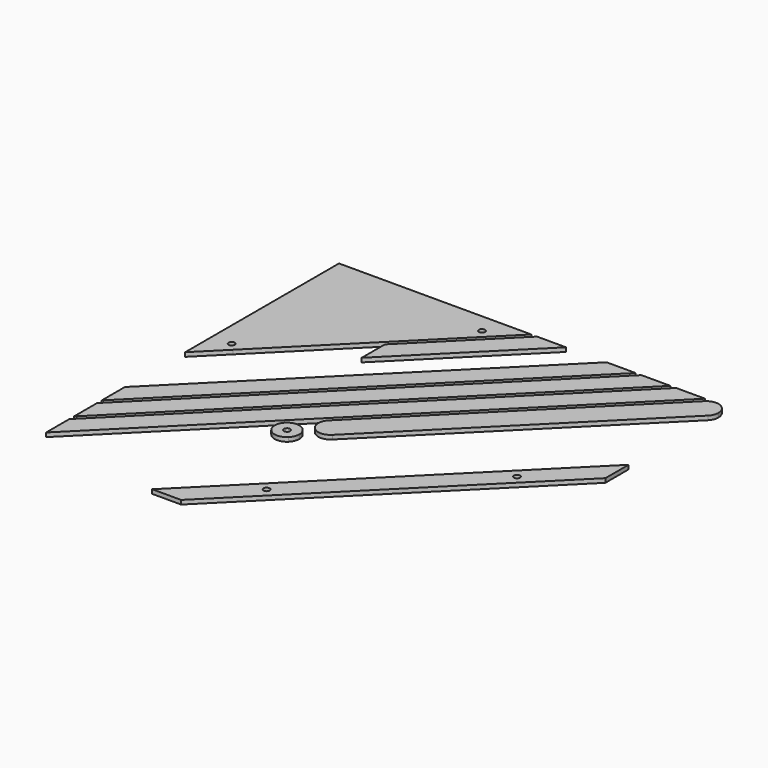
from build123d import *

# Parameters (mm, degrees)
F0_R     = 9.525
F1_DEPTH = 6.35


with BuildPart() as f1:
    # F0 (on Top) → F1 (new body, symmetric)
    with BuildSketch(Plane.XY):
        Polygon((-115.17049, 603.25), (-603.25, 603.25), (-603.25, 97.209977), (-603.25, 7.407416), (-520.854856, 89.802561), (-89.802561, 520.854855), (-7.407416, 603.25), align=None)
        with BuildLine():
            ThreePointArc((-511.555495, 112.253202), (-513.97232, 100.103002), (-520.854856, 89.802561))
            ThreePointArc((-520.854856, 89.802561), (-572.63867, 124.403401), (-511.555495, 112.253202))
        make_face(mode=Mode.SUBTRACT)
        with BuildLine():
            ThreePointArc((-80.503202, 543.305495), (-82.920026, 531.155296), (-89.802561, 520.854855))
            ThreePointArc((-89.802561, 520.854855), (-141.586377, 555.455694), (-80.503202, 543.305495))
        make_face(mode=Mode.SUBTRACT)
        with BuildLine():
            ThreePointArc((-511.555495, 112.253202), (-572.63867, 124.403401), (-520.854856, 89.802561))
            ThreePointArc((-520.854856, 89.802561), (-513.97232, 100.103002), (-511.555495, 112.253202))
        make_face()
        with Locations((-543.305495, 112.253202)):
            Circle(F0_R, mode=Mode.SUBTRACT)
        with BuildLine():
            ThreePointArc((-80.503202, 543.305495), (-141.586377, 555.455694), (-89.802561, 520.854855))
            ThreePointArc((-89.802561, 520.854855), (-82.920026, 531.155296), (-80.503202, 543.305495))
        make_face()
        with Locations((-112.253202, 543.305495)):
            Circle(F0_R, mode=Mode.SUBTRACT)
    extrude(amount=F1_DEPTH, both=True)


with BuildPart() as f1b:
    # F0 (on Top) → F1, piece 2 (new body, symmetric)
    with BuildSketch(Plane.XY):
        Polygon((-603.25, -226.079243), (-603.25, -315.881804), (-178.032283, 109.335913), (-222.933563, 154.237194), align=None)
        Polygon((-222.933563, 154.237194), (-178.032283, 109.335913), (315.881804, 603.25), (226.079243, 603.25), align=None)
    extrude(amount=F1_DEPTH, both=True)


with BuildPart() as f1c:
    # F0 (on Top) → F1, piece 3 (new body, symmetric)
    with BuildSketch(Plane.XY):
        Polygon((333.842316, 603.25), (-603.25, -333.842316), (-603.25, -423.644878), (423.644878, 603.25), align=None)
    extrude(amount=F1_DEPTH, both=True)


with BuildPart() as f1d:
    # F0 (on Top) → F1, piece 4 (new body, symmetric)
    with BuildSketch(Plane.XY):
        Polygon((-603.25, -441.60539), (-603.25, -531.407951), (531.407951, 603.25), (441.60539, 603.25), align=None)
    extrude(amount=F1_DEPTH, both=True)


with BuildPart() as f1e:
    # F0 (on Top) → F1, piece 5 (new body, symmetric)
    with BuildSketch(Plane.XY):
        with BuildLine():
            ThreePointArc((592.090768, 592.090768), (579.730239, 600.34981), (565.15, 603.25))
            ThreePointArc((565.15, 603.25), (550.569761, 600.34981), (538.209232, 592.090768))
            Line((538.209232, 592.090768), (-108.369209, -54.487672))
            ThreePointArc((-108.369209, -54.487672), (-119.528441, -81.428441), (-108.369209, -108.369209))
            Line((-108.369209, -108.369209), (592.090768, 592.090768))
        make_face()
        with BuildLine():
            ThreePointArc((592.090768, 538.209232), (600.34981, 550.569761), (603.25, 565.15))
            ThreePointArc((603.25, 565.15), (600.34981, 579.730239), (592.090768, 592.090768))
            Line((592.090768, 592.090768), (-108.369209, -108.369209))
            ThreePointArc((-108.369209, -108.369209), (-81.428441, -119.528441), (-54.487672, -108.369209))
            Line((-54.487672, -108.369209), (592.090768, 538.209232))
        make_face()
    extrude(amount=F1_DEPTH, both=True)


with BuildPart() as f1f:
    # F0 (on Top) → F1, piece 6 (new body, symmetric)
    with BuildSketch(Plane.XY):
        with BuildLine():
            ThreePointArc((-118.448346, -156.548346), (-121.348536, -141.968108), (-129.607578, -129.607578))
            Line((-129.607578, -129.607578), (-149.835105, -149.835105))
            ThreePointArc((-149.835105, -149.835105), (-147.346205, -153.098955), (-146.461831, -157.1071))
            ThreePointArc((-146.461831, -157.1071), (-152.711172, -166.051131), (-163.258825, -163.258825))
            Line((-163.258825, -163.258825), (-183.489115, -183.489115))
            ThreePointArc((-183.489115, -183.489115), (-156.548347, -194.648346), (-129.607578, -183.489115))
            ThreePointArc((-129.607578, -183.489115), (-121.348536, -171.128585), (-118.448346, -156.548346))
        make_face()
        with BuildLine():
            Line((-149.835105, -149.835105), (-129.607578, -129.607578))
            ThreePointArc((-129.607578, -129.607578), (-156.548347, -118.448346), (-183.489116, -129.607579))
            ThreePointArc((-183.489116, -129.607579), (-194.648346, -156.548347), (-183.489115, -183.489115))
            Line((-183.489115, -183.489115), (-163.258825, -163.258825))
            ThreePointArc((-163.258825, -163.258825), (-162.722023, -150.371908), (-149.835105, -149.835105))
        make_face()
    extrude(amount=F1_DEPTH, both=True)


with BuildPart() as f1g:
    # F0 (on Top) → F1, piece 7 (new body, symmetric)
    with BuildSketch(Plane.XY):
        with BuildLine():
            Line((-22.45064, -408.601654), (-217.098987, -603.25))
            Line((-217.098987, -603.25), (-127.296426, -603.25))
            Line((-127.296426, -603.25), (22.45064, -453.502934))
            ThreePointArc((22.45064, -453.502934), (-22.45064, -453.502934), (-22.45064, -408.601654))
        make_face()
        with BuildLine():
            Line((408.601653, 22.45064), (-22.45064, -408.601654))
            ThreePointArc((-22.45064, -408.601654), (12.150199, -401.719119), (31.75, -431.052294))
            ThreePointArc((31.75, -431.052294), (29.333175, -443.202493), (22.45064, -453.502934))
            Line((22.45064, -453.502934), (453.502934, -22.45064))
            ThreePointArc((453.502934, -22.45064), (408.601654, -22.450641), (408.601653, 22.45064))
        make_face()
        with BuildLine():
            Line((603.25, 217.098987), (408.601653, 22.45064))
            ThreePointArc((408.601653, 22.45064), (443.202492, 29.333175), (462.802294, 0))
            ThreePointArc((462.802294, 0), (460.385469, -12.150199), (453.502934, -22.45064))
            Line((453.502934, -22.45064), (603.25, 127.296426))
            Line((603.25, 127.296426), (603.25, 217.098987))
        make_face()
        with BuildLine():
            ThreePointArc((31.75, -431.052294), (12.150199, -401.719119), (-22.45064, -408.601654))
            ThreePointArc((-22.45064, -408.601654), (-22.45064, -453.502934), (22.45064, -453.502934))
            ThreePointArc((22.45064, -453.502934), (29.333175, -443.202493), (31.75, -431.052294))
        make_face()
        with Locations((0, -431.052294)):
            Circle(F0_R, mode=Mode.SUBTRACT)
        with BuildLine():
            ThreePointArc((462.802294, 0), (443.202492, 29.333175), (408.601653, 22.45064))
            ThreePointArc((408.601653, 22.45064), (408.601654, -22.450641), (453.502934, -22.45064))
            ThreePointArc((453.502934, -22.45064), (460.385469, -12.150199), (462.802294, 0))
        make_face()
        with Locations((431.052294, 0)):
            Circle(F0_R, mode=Mode.SUBTRACT)
    extrude(amount=F1_DEPTH, both=True)


with BuildPart() as f1h:
    # F0 (on Top) → F1, piece 8 (new body, symmetric)
    with BuildSketch(Plane.XY):
        Polygon((-251.447171, 341.249733), (-251.447171, 251.447171), (100.355657, 603.25), (10.553096, 603.25), align=None)
    extrude(amount=F1_DEPTH, both=True)


solid = Compound([f1.part, f1b.part, f1c.part, f1d.part, f1e.part, f1f.part, f1g.part, f1h.part])
